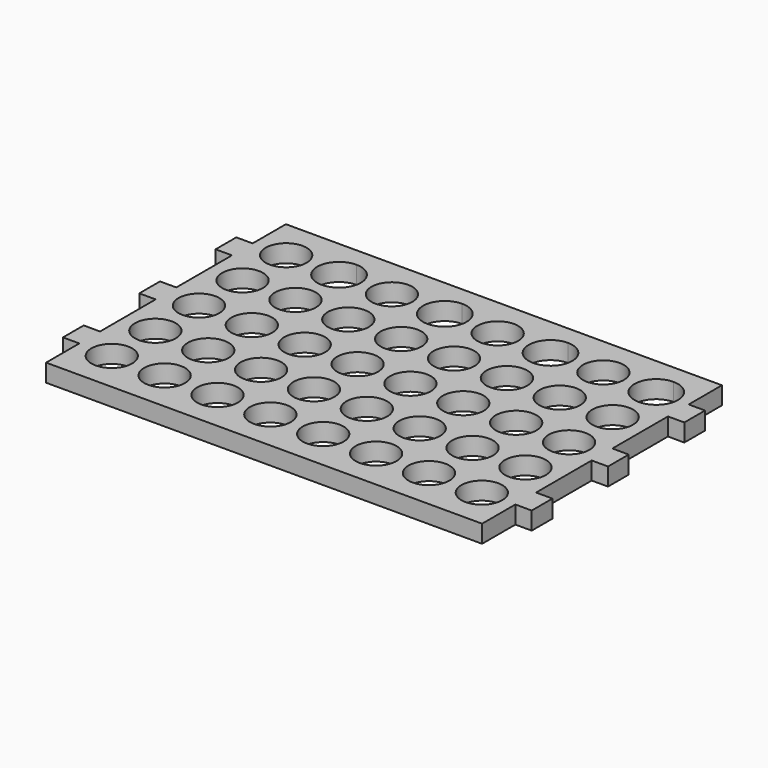
from build123d import *

# Parameters (mm, degrees)
F0_W     = 160
F0_H     = 110
F1_DEPTH = 6.5
F3_DEPTH = 6
F5_DEPTH = 6
F7_DEPTH = 25


# Not quite as in the source:
# - a feature names something its author has since deleted; it is built from what else it names


with BuildPart() as f1:
    # F0 (on Top) → F1 (new body)
    with BuildSketch(Plane.XY):
        Rectangle(F0_W, F0_H)
    extrude(amount=F1_DEPTH)

    # F2 (on face) → F3 (join)
    with BuildSketch(Plane(origin=(-80, 0, 0), x_dir=(0, -1, 0), z_dir=(-1, 0, 0))):
        Polygon((-39.75, 6.5), (-39.75, 3.25), (-35, 3.25), (-30.25, 3.25), (-30.25, 6.5), align=None)
        Polygon((-35, 3.25), (-39.75, 3.25), (-39.75, 0), (-30.25, 0), (-30.25, 3.25), align=None)
        Polygon((-4.75, 6.5), (-4.75, 3.25), (0, 3.25), (4.75, 3.25), (4.75, 6.5), align=None)
        Polygon((0, 3.25), (-4.75, 3.25), (-4.75, 0), (4.75, 0), (4.75, 3.25), align=None)
        Polygon((39.75, 6.5), (30.25, 6.5), (30.25, 3.25), (35, 3.25), (39.75, 3.25), align=None)
        Polygon((30.25, 3.25), (30.25, 0), (39.75, 0), (39.75, 3.25), (35, 3.25), align=None)
    extrude(amount=F3_DEPTH)

    # F4 (on face) → F5 (join)
    with BuildSketch(Plane.YZ.offset(80)):
        Polygon((-39.75, 6.5), (-39.75, 3.25), (-35, 3.25), (-30.25, 3.25), (-30.25, 6.5), align=None)
        Polygon((-35, 3.25), (-39.75, 3.25), (-39.75, 0), (-30.25, 0), (-30.25, 3.25), align=None)
        Polygon((-4.75, 6.5), (-4.75, 3.25), (0, 3.25), (4.75, 3.25), (4.75, 6.5), align=None)
        Polygon((0, 3.25), (-4.75, 3.25), (-4.75, 0), (4.75, 0), (4.75, 3.25), align=None)
        Polygon((39.75, 6.5), (30.25, 6.5), (30.25, 3.25), (30.25, 0), (39.75, 0), align=None)
    extrude(amount=F5_DEPTH)

    # F6 (on face) → F7 (cut)
    with BuildSketch(Plane.XY.offset(6.5)):
        with BuildLine():
            Line((-67.9, 40), (-67.9, 47.5))
            ThreePointArc((-67.9, 47.5), (-75.4, 40), (-67.9, 32.5))
            Line((-67.9, 32.5), (-67.9, 40))
        make_face()
        with BuildLine():
            ThreePointArc((-60.4, 40), (-62.5966991411, 45.3033008589), (-67.9, 47.5))
            Line((-67.9, 47.5), (-67.9, 40))
            Line((-67.9, 40), (-67.9, 32.5))
            ThreePointArc((-67.9, 32.5), (-62.5966991411, 34.6966991411), (-60.4, 40))
        make_face()
        with BuildLine():
            Line((-48.5, 32.0100222161), (-48.5, 47.9899777839))
            ThreePointArc((-48.5, 47.9899777839), (-56.4899777839, 40), (-48.5, 32.0100222161))
        make_face()
        with BuildLine():
            ThreePointArc((-40.5100222161, 40), (-42.8502325275, 45.6497674725), (-48.5, 47.9899777839))
            Line((-48.5, 47.9899777839), (-48.5, 32.0100222161))
            ThreePointArc((-48.5, 32.0100222161), (-42.8502325275, 34.3502325275), (-40.5100222161, 40))
        make_face()
        with BuildLine():
            Line((-29.1, 32.5), (-29.1, 47.5))
            ThreePointArc((-29.1, 47.5), (-36.6, 40), (-29.1, 32.5))
        make_face()
        with BuildLine():
            ThreePointArc((-21.6, 40), (-23.7966991411, 45.3033008589), (-29.1, 47.5))
            Line((-29.1, 47.5), (-29.1, 32.5))
            ThreePointArc((-29.1, 32.5), (-23.7966991411, 34.6966991411), (-21.6, 40))
        make_face()
        with BuildLine():
            Line((-9.7, 32.0100222161), (-9.7, 47.9899777839))
            ThreePointArc((-9.7, 47.9899777839), (-17.6899777839, 40), (-9.7, 32.0100222161))
        make_face()
        with BuildLine():
            ThreePointArc((-1.7100222161, 40), (-4.0502325275, 45.6497674725), (-9.7, 47.9899777839))
            Line((-9.7, 47.9899777839), (-9.7, 32.0100222161))
            ThreePointArc((-9.7, 32.0100222161), (-4.0502325275, 34.3502325275), (-1.7100222161, 40))
        make_face()
        with BuildLine():
            Line((9.7, 32.5), (9.7, 47.5))
            ThreePointArc((9.7, 47.5), (2.2, 40), (9.7, 32.5))
        make_face()
        with BuildLine():
            ThreePointArc((17.2, 40), (15.0033008589, 45.3033008589), (9.7, 47.5))
            Line((9.7, 47.5), (9.7, 32.5))
            ThreePointArc((9.7, 32.5), (15.0033008589, 34.6966991411), (17.2, 40))
        make_face()
        with BuildLine():
            Line((29.1, 32.0100222161), (29.1, 47.9899777839))
            ThreePointArc((29.1, 47.9899777839), (21.1100222161, 40), (29.1, 32.0100222161))
        make_face()
        with BuildLine():
            ThreePointArc((37.0899777839, 40), (34.7497674725, 45.6497674725), (29.1, 47.9899777839))
            Line((29.1, 47.9899777839), (29.1, 32.0100222161))
            ThreePointArc((29.1, 32.0100222161), (34.7497674725, 34.3502325275), (37.0899777839, 40))
        make_face()
        with BuildLine():
            Line((48.5, 32.5), (48.5, 47.5))
            ThreePointArc((48.5, 47.5), (41, 40), (48.5, 32.5))
        make_face()
        with BuildLine():
            ThreePointArc((56, 40), (53.8033008589, 45.3033008589), (48.5, 47.5))
            Line((48.5, 47.5), (48.5, 32.5))
            ThreePointArc((48.5, 32.5), (53.8033008589, 34.6966991411), (56, 40))
        make_face()
        with BuildLine():
            Line((67.9, 32.0100222161), (67.9, 47.9899777839))
            ThreePointArc((67.9, 47.9899777839), (59.9100222161, 40), (67.9, 32.0100222161))
        make_face()
        with BuildLine():
            ThreePointArc((75.8899777839, 40), (73.5497674725, 45.6497674725), (67.9, 47.9899777839))
            Line((67.9, 47.9899777839), (67.9, 32.0100222161))
            ThreePointArc((67.9, 32.0100222161), (73.5497674725, 34.3502325275), (75.8899777839, 40))
        make_face()
        with BuildLine():
            ThreePointArc((75.4, 20), (73.2033008589, 25.3033008589), (67.9, 27.5))
            Line((67.9, 27.5), (67.9, 12.5))
            ThreePointArc((67.9, 12.5), (73.2033008589, 14.6966991411), (75.4, 20))
        make_face()
        with BuildLine():
            Line((67.9, 12.5), (67.9, 27.5))
            ThreePointArc((67.9, 27.5), (60.4, 20), (67.9, 12.5))
        make_face()
        with BuildLine():
            ThreePointArc((56, 20), (53.8033008589, 25.3033008589), (48.5, 27.5))
            Line((48.5, 27.5), (48.5, 12.5))
            ThreePointArc((48.5, 12.5), (53.8033008589, 14.6966991411), (56, 20))
        make_face()
        with BuildLine():
            Line((48.5, 12.5), (48.5, 27.5))
            ThreePointArc((48.5, 27.5), (41, 20), (48.5, 12.5))
        make_face()
        with BuildLine():
            ThreePointArc((36.6, 20), (34.4033008589, 25.3033008589), (29.1, 27.5))
            Line((29.1, 27.5), (29.1, 12.5))
            ThreePointArc((29.1, 12.5), (34.4033008589, 14.6966991411), (36.6, 20))
        make_face()
        with BuildLine():
            Line((29.1, 12.5), (29.1, 27.5))
            ThreePointArc((29.1, 27.5), (21.6, 20), (29.1, 12.5))
        make_face()
        with BuildLine():
            ThreePointArc((17.2, 20), (15.0033008589, 25.3033008589), (9.7, 27.5))
            Line((9.7, 27.5), (9.7, 12.5))
            ThreePointArc((9.7, 12.5), (15.0033008589, 14.6966991411), (17.2, 20))
        make_face()
        with BuildLine():
            Line((9.7, 12.5), (9.7, 27.5))
            ThreePointArc((9.7, 27.5), (2.2, 20), (9.7, 12.5))
        make_face()
        with BuildLine():
            ThreePointArc((-2.2, 20), (-4.3966991411, 25.3033008589), (-9.7, 27.5))
            Line((-9.7, 27.5), (-9.7, 12.5))
            ThreePointArc((-9.7, 12.5), (-4.3966991411, 14.6966991411), (-2.2, 20))
        make_face()
        with BuildLine():
            Line((-9.7, 12.5), (-9.7, 27.5))
            ThreePointArc((-9.7, 27.5), (-17.2, 20), (-9.7, 12.5))
        make_face()
        with BuildLine():
            ThreePointArc((-21.6, 20), (-23.7966991411, 25.3033008589), (-29.1, 27.5))
            Line((-29.1, 27.5), (-29.1, 12.5))
            ThreePointArc((-29.1, 12.5), (-23.7966991411, 14.6966991411), (-21.6, 20))
        make_face()
        with BuildLine():
            Line((-29.1, 12.5), (-29.1, 27.5))
            ThreePointArc((-29.1, 27.5), (-36.6, 20), (-29.1, 12.5))
        make_face()
        with BuildLine():
            ThreePointArc((-41, 20), (-43.1966991411, 25.3033008589), (-48.5, 27.5))
            Line((-48.5, 27.5), (-48.5, 12.5))
            ThreePointArc((-48.5, 12.5), (-43.1966991411, 14.6966991411), (-41, 20))
        make_face()
        with BuildLine():
            Line((-48.5, 12.5), (-48.5, 27.5))
            ThreePointArc((-48.5, 27.5), (-56, 20), (-48.5, 12.5))
        make_face()
        with BuildLine():
            ThreePointArc((-60.4, 20), (-62.5966991411, 25.3033008589), (-67.9, 27.5))
            Line((-67.9, 27.5), (-67.9, 20))
            Line((-67.9, 20), (-67.9, 12.5))
            ThreePointArc((-67.9, 12.5), (-62.5966991411, 14.6966991411), (-60.4, 20))
        make_face()
        with BuildLine():
            Line((-67.9, 20), (-67.9, 27.5))
            ThreePointArc((-67.9, 27.5), (-75.4, 20), (-67.9, 12.5))
            Line((-67.9, 12.5), (-67.9, 20))
        make_face()
        with BuildLine():
            Line((-67.9, 0), (-67.9, 7.5))
            ThreePointArc((-67.9, 7.5), (-75.4, 0), (-67.9, -7.5))
            Line((-67.9, -7.5), (-67.9, 0))
        make_face()
        with BuildLine():
            ThreePointArc((-60.4, 0), (-62.5966991411, 5.3033008589), (-67.9, 7.5))
            Line((-67.9, 7.5), (-67.9, 0))
            Line((-67.9, 0), (-67.9, -7.5))
            ThreePointArc((-67.9, -7.5), (-62.5966991411, -5.3033008589), (-60.4, 0))
        make_face()
        with BuildLine():
            Line((-48.5, -7.5), (-48.5, 7.5))
            ThreePointArc((-48.5, 7.5), (-56, 0), (-48.5, -7.5))
        make_face()
        with BuildLine():
            ThreePointArc((-41, 0), (-43.1966991411, 5.3033008589), (-48.5, 7.5))
            Line((-48.5, 7.5), (-48.5, -7.5))
            ThreePointArc((-48.5, -7.5), (-43.1966991411, -5.3033008589), (-41, 0))
        make_face()
        with BuildLine():
            Line((-29.1, -7.5), (-29.1, 7.5))
            ThreePointArc((-29.1, 7.5), (-36.6, 0), (-29.1, -7.5))
        make_face()
        with BuildLine():
            ThreePointArc((-21.6, 0), (-23.7966991411, 5.3033008589), (-29.1, 7.5))
            Line((-29.1, 7.5), (-29.1, -7.5))
            ThreePointArc((-29.1, -7.5), (-23.7966991411, -5.3033008589), (-21.6, 0))
        make_face()
        with BuildLine():
            Line((-9.7, -7.5), (-9.7, 7.5))
            ThreePointArc((-9.7, 7.5), (-17.2, 0), (-9.7, -7.5))
        make_face()
        with BuildLine():
            ThreePointArc((-2.2, 0), (-4.3966991411, 5.3033008589), (-9.7, 7.5))
            Line((-9.7, 7.5), (-9.7, -7.5))
            ThreePointArc((-9.7, -7.5), (-4.3966991411, -5.3033008589), (-2.2, 0))
        make_face()
        with BuildLine():
            Line((9.7, -7.5), (9.7, 7.5))
            ThreePointArc((9.7, 7.5), (2.2, 0), (9.7, -7.5))
        make_face()
        with BuildLine():
            ThreePointArc((17.2, 0), (15.0033008589, 5.3033008589), (9.7, 7.5))
            Line((9.7, 7.5), (9.7, -7.5))
            ThreePointArc((9.7, -7.5), (15.0033008589, -5.3033008589), (17.2, 0))
        make_face()
        with BuildLine():
            Line((29.1, -7.5), (29.1, 7.5))
            ThreePointArc((29.1, 7.5), (21.6, 0), (29.1, -7.5))
        make_face()
        with BuildLine():
            ThreePointArc((36.6, 0), (34.4033008589, 5.3033008589), (29.1, 7.5))
            Line((29.1, 7.5), (29.1, -7.5))
            ThreePointArc((29.1, -7.5), (34.4033008589, -5.3033008589), (36.6, 0))
        make_face()
        with BuildLine():
            Line((48.5, -7.5), (48.5, 7.5))
            ThreePointArc((48.5, 7.5), (41, 0), (48.5, -7.5))
        make_face()
        with BuildLine():
            ThreePointArc((56, 0), (53.8033008589, 5.3033008589), (48.5, 7.5))
            Line((48.5, 7.5), (48.5, -7.5))
            ThreePointArc((48.5, -7.5), (53.8033008589, -5.3033008589), (56, 0))
        make_face()
        with BuildLine():
            Line((67.9, -7.5), (67.9, 7.5))
            ThreePointArc((67.9, 7.5), (60.4, 0), (67.9, -7.5))
        make_face()
        with BuildLine():
            ThreePointArc((75.4, 0), (73.2033008589, 5.3033008589), (67.9, 7.5))
            Line((67.9, 7.5), (67.9, -7.5))
            ThreePointArc((67.9, -7.5), (73.2033008589, -5.3033008589), (75.4, 0))
        make_face()
        with BuildLine():
            ThreePointArc((75.4, -20), (73.2033008589, -14.6966991411), (67.9, -12.5))
            Line((67.9, -12.5), (67.9, -27.5))
            ThreePointArc((67.9, -27.5), (73.2033008589, -25.3033008589), (75.4, -20))
        make_face()
        with BuildLine():
            Line((67.9, -27.5), (67.9, -12.5))
            ThreePointArc((67.9, -12.5), (60.4, -20), (67.9, -27.5))
        make_face()
        with BuildLine():
            ThreePointArc((56, -20), (53.8033008589, -14.6966991411), (48.5, -12.5))
            Line((48.5, -12.5), (48.5, -27.5))
            ThreePointArc((48.5, -27.5), (53.8033008589, -25.3033008589), (56, -20))
        make_face()
        with BuildLine():
            Line((48.5, -27.5), (48.5, -12.5))
            ThreePointArc((48.5, -12.5), (41, -20), (48.5, -27.5))
        make_face()
        with BuildLine():
            ThreePointArc((36.6, -20), (34.4033008589, -14.6966991411), (29.1, -12.5))
            Line((29.1, -12.5), (29.1, -27.5))
            ThreePointArc((29.1, -27.5), (34.4033008589, -25.3033008589), (36.6, -20))
        make_face()
        with BuildLine():
            Line((29.1, -27.5), (29.1, -12.5))
            ThreePointArc((29.1, -12.5), (21.6, -20), (29.1, -27.5))
        make_face()
        with BuildLine():
            ThreePointArc((17.2, -20), (15.0033008589, -14.6966991411), (9.7, -12.5))
            Line((9.7, -12.5), (9.7, -27.5))
            ThreePointArc((9.7, -27.5), (15.0033008589, -25.3033008589), (17.2, -20))
        make_face()
        with BuildLine():
            Line((9.7, -27.5), (9.7, -12.5))
            ThreePointArc((9.7, -12.5), (2.2, -20), (9.7, -27.5))
        make_face()
        with BuildLine():
            ThreePointArc((-2.2, -20), (-4.3966991411, -14.6966991411), (-9.7, -12.5))
            Line((-9.7, -12.5), (-9.7, -27.5))
            ThreePointArc((-9.7, -27.5), (-4.3966991411, -25.3033008589), (-2.2, -20))
        make_face()
        with BuildLine():
            Line((-9.7, -27.5), (-9.7, -12.5))
            ThreePointArc((-9.7, -12.5), (-17.2, -20), (-9.7, -27.5))
        make_face()
        with BuildLine():
            ThreePointArc((-21.6, -20), (-23.7966991411, -14.6966991411), (-29.1, -12.5))
            Line((-29.1, -12.5), (-29.1, -27.5))
            ThreePointArc((-29.1, -27.5), (-23.7966991411, -25.3033008589), (-21.6, -20))
        make_face()
        with BuildLine():
            Line((-29.1, -27.5), (-29.1, -12.5))
            ThreePointArc((-29.1, -12.5), (-36.6, -20), (-29.1, -27.5))
        make_face()
        with BuildLine():
            ThreePointArc((-41, -20), (-43.1966991411, -14.6966991411), (-48.5, -12.5))
            Line((-48.5, -12.5), (-48.5, -27.5))
            ThreePointArc((-48.5, -27.5), (-43.1966991411, -25.3033008589), (-41, -20))
        make_face()
        with BuildLine():
            Line((-48.5, -27.5), (-48.5, -12.5))
            ThreePointArc((-48.5, -12.5), (-56, -20), (-48.5, -27.5))
        make_face()
        with BuildLine():
            ThreePointArc((-60.4, -20), (-62.5966991411, -14.6966991411), (-67.9, -12.5))
            Line((-67.9, -12.5), (-67.9, -20))
            Line((-67.9, -20), (-67.9, -27.5))
            ThreePointArc((-67.9, -27.5), (-62.5966991411, -25.3033008589), (-60.4, -20))
        make_face()
        with BuildLine():
            Line((-67.9, -20), (-67.9, -12.5))
            ThreePointArc((-67.9, -12.5), (-75.4, -20), (-67.9, -27.5))
            Line((-67.9, -27.5), (-67.9, -20))
        make_face()
        with BuildLine():
            ThreePointArc((-60.4, -40), (-62.5966991411, -34.6966991411), (-67.9, -32.5))
            ThreePointArc((-67.9, -32.5), (-73.2033008589, -45.3033008589), (-60.4, -40))
        make_face()
        with BuildLine():
            Line((-48.5, -47.5), (-48.5, -32.5))
            ThreePointArc((-48.5, -32.5), (-56, -40), (-48.5, -47.5))
        make_face()
        with BuildLine():
            ThreePointArc((-41, -40), (-43.1966991411, -34.6966991411), (-48.5, -32.5))
            Line((-48.5, -32.5), (-48.5, -47.5))
            ThreePointArc((-48.5, -47.5), (-43.1966991411, -45.3033008589), (-41, -40))
        make_face()
        with BuildLine():
            Line((-29.1, -47.5), (-29.1, -32.5))
            ThreePointArc((-29.1, -32.5), (-36.6, -40), (-29.1, -47.5))
        make_face()
        with BuildLine():
            ThreePointArc((-21.6, -40), (-23.7966991411, -34.6966991411), (-29.1, -32.5))
            Line((-29.1, -32.5), (-29.1, -47.5))
            ThreePointArc((-29.1, -47.5), (-23.7966991411, -45.3033008589), (-21.6, -40))
        make_face()
        with BuildLine():
            Line((-9.7, -47.5), (-9.7, -32.5))
            ThreePointArc((-9.7, -32.5), (-17.2, -40), (-9.7, -47.5))
        make_face()
        with BuildLine():
            ThreePointArc((-2.2, -40), (-4.3966991411, -34.6966991411), (-9.7, -32.5))
            Line((-9.7, -32.5), (-9.7, -47.5))
            ThreePointArc((-9.7, -47.5), (-4.3966991411, -45.3033008589), (-2.2, -40))
        make_face()
        with BuildLine():
            Line((9.7, -47.5), (9.7, -32.5))
            ThreePointArc((9.7, -32.5), (2.2, -40), (9.7, -47.5))
        make_face()
        with BuildLine():
            ThreePointArc((17.2, -40), (15.0033008589, -34.6966991411), (9.7, -32.5))
            Line((9.7, -32.5), (9.7, -47.5))
            ThreePointArc((9.7, -47.5), (15.0033008589, -45.3033008589), (17.2, -40))
        make_face()
        with BuildLine():
            Line((29.1, -47.5), (29.1, -32.5))
            ThreePointArc((29.1, -32.5), (21.6, -40), (29.1, -47.5))
        make_face()
        with BuildLine():
            ThreePointArc((36.6, -40), (34.4033008589, -34.6966991411), (29.1, -32.5))
            Line((29.1, -32.5), (29.1, -47.5))
            ThreePointArc((29.1, -47.5), (34.4033008589, -45.3033008589), (36.6, -40))
        make_face()
        with BuildLine():
            Line((48.5, -47.5), (48.5, -32.5))
            ThreePointArc((48.5, -32.5), (41, -40), (48.5, -47.5))
        make_face()
        with BuildLine():
            ThreePointArc((56, -40), (53.8033008589, -34.6966991411), (48.5, -32.5))
            Line((48.5, -32.5), (48.5, -47.5))
            ThreePointArc((48.5, -47.5), (53.8033008589, -45.3033008589), (56, -40))
        make_face()
        with BuildLine():
            Line((67.9, -47.5), (67.9, -32.5))
            ThreePointArc((67.9, -32.5), (60.4, -40), (67.9, -47.5))
        make_face()
        with BuildLine():
            ThreePointArc((75.4, -40), (73.2033008589, -34.6966991411), (67.9, -32.5))
            Line((67.9, -32.5), (67.9, -47.5))
            ThreePointArc((67.9, -47.5), (73.2033008589, -45.3033008589), (75.4, -40))
        make_face()
    extrude(amount=-F7_DEPTH, mode=Mode.SUBTRACT)


solid = f1.part
